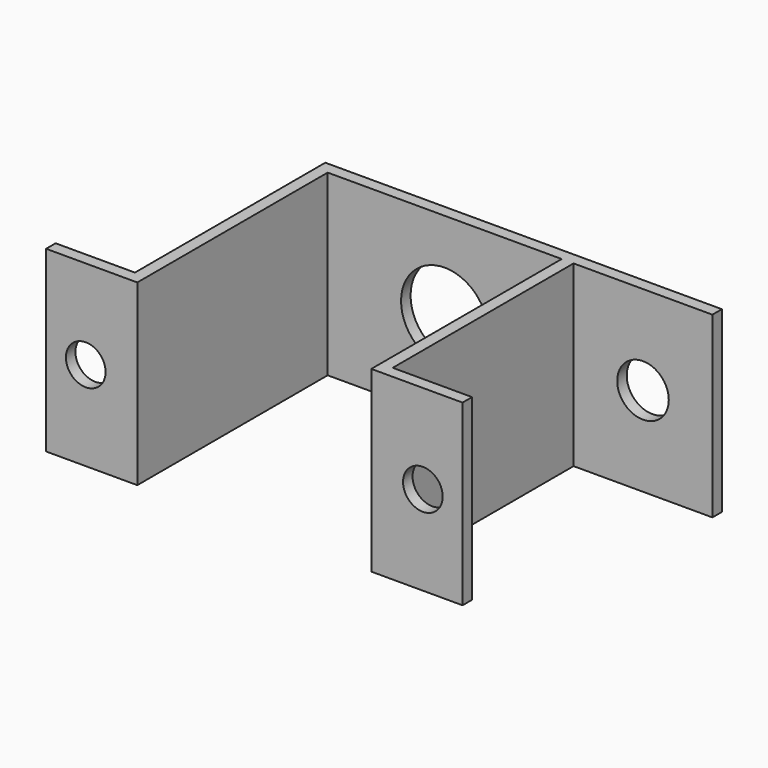
from build123d import *

# Parameters (mm, degrees)
F0_W           = 20
F0_H           = 3
F2_DEPTH       = 22.5
F3_D           = 13
F3_DEPTH       = 10
F3_TIP         = 3.9055940237
F4_D           = 22
F4_DEPTH       = 10
F4_TIP         = 6.6094668093
F7_D           = 10
F7_DEPTH       = 10
F7_TIP         = 3.0043030951
F7_ON_F5_D     = 10
F7_ON_F5_DEPTH = 10
F7_ON_F5_TIP   = 3.0043030951


# Not quite as in the source:
# - a feature names something its author has since deleted; it is built from what else it names


with BuildPart() as f2:
    # F0 (on Top) → F2 (new body, symmetric)
    with BuildSketch(Plane.XY):
        Polygon((-47, 0), (0, 0), (12, 0), (15, 0), (50, 0), (50, 3), (-50, 3), (-50, 0), align=None)
        Polygon((15, 0), (12, 0), (12, -60), (15, -60), (15, -57), align=None)
        Polygon((-47, -60), (-47, 0), (-50, 0), (-50, -57), (-50, -60), align=None)
        with Locations((-60, -58.5)):
            Rectangle(F0_W, F0_H)
        with Locations((25, -58.5)):
            Rectangle(F0_W, F0_H)
    extrude(amount=F2_DEPTH, both=True)

    # F3 (one way)
    with BuildSketch(Plane.XZ):
        with Locations((32.5, 0)):
            Circle(F3_D / 2)
    extrude(amount=-F3_DEPTH, mode=Mode.SUBTRACT)
    with Locations(Plane.XZ):
        with Locations((32.5, 0)):
            with Locations((0, 0, -(F3_DEPTH + F3_TIP / 2))):  # 118° drill point
                Cone(0, F3_D / 2, F3_TIP, mode=Mode.SUBTRACT)

    # F4
    with Locations(Plane.XZ):
        with Locations((-17.5, 0)):
            Hole(F4_D / 2, depth=F4_DEPTH)
            with Locations((0, 0, -(F4_DEPTH + F4_TIP / 2))):  # 118° drill point
                Cone(0, F4_D / 2, F4_TIP, mode=Mode.SUBTRACT)

    # F7 (one way)
    with BuildSketch(Plane(origin=(0, -57, 0), x_dir=(-1, 0, 0), z_dir=(0, 1, 0))):
        with Locations((-25, 0)):
            Circle(F7_D / 2)
    extrude(amount=-F7_DEPTH, mode=Mode.SUBTRACT)
    with Locations(Plane(origin=(0, -57, 0), x_dir=(-1, 0, 0), z_dir=(0, 1, 0))):
        with Locations((-25, 0)):
            with Locations((0, 0, -(F7_DEPTH + F7_TIP / 2))):  # 118° drill point
                Cone(0, F7_D / 2, F7_TIP, mode=Mode.SUBTRACT)

    # F7 on F5
    with Locations(Plane(origin=(0, -57, 0), x_dir=(-1, 0, 0), z_dir=(0, 1, 0))):
        with Locations((60, 0)):
            Hole(F7_ON_F5_D / 2, depth=F7_ON_F5_DEPTH)
            with Locations((0, 0, -(F7_ON_F5_DEPTH + F7_ON_F5_TIP / 2))):  # 118° drill point
                Cone(0, F7_ON_F5_D / 2, F7_ON_F5_TIP, mode=Mode.SUBTRACT)


solid = f2.part
